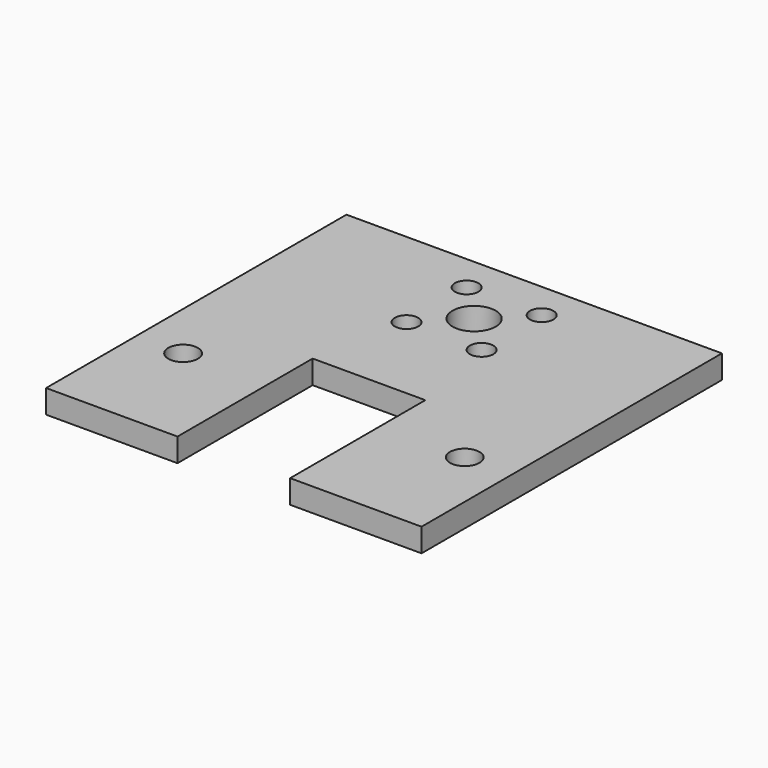
from build123d import *

# Parameters (mm, degrees)
F0_R     = 2
F0_R_2   = 1.5875
F0_R_3   = 2.921
F1_DEPTH = 3.175


# Not quite as in the source:
# - a feature names something its author has since deleted; it is built from what else it names


with BuildPart() as f1:
    # F0 (on Top) → F1 (new body)
    with BuildSketch(Plane.XY):
        Polygon((-25.4, 76.2436284547), (-25.4, 25.4436284547), (-7.62, 25.4436284547), (-7.62, 48.3036284547), (7.62, 48.3036284547), (7.62, 25.4436284547), (25.4, 25.4436284547), (25.4, 76.2436284547), align=None)
        with Locations((-19.05, 40.6836284547)):
            Circle(F0_R, mode=Mode.SUBTRACT)
        with Locations((19.05, 40.6836284547)):
            Circle(F0_R, mode=Mode.SUBTRACT)
        with Locations((-5.08, 61.0036284547)):
            Circle(F0_R_2, mode=Mode.SUBTRACT)
        with Locations((0, 66.0836284547)):
            Circle(F0_R_3, mode=Mode.SUBTRACT)
        with Locations((-5.08, 71.1636284547)):
            Circle(F0_R_2, mode=Mode.SUBTRACT)
        with Locations((5.08, 61.0036284547)):
            Circle(F0_R_2, mode=Mode.SUBTRACT)
        with Locations((5.08, 71.1636284547)):
            Circle(F0_R_2, mode=Mode.SUBTRACT)
    extrude(amount=F1_DEPTH)


solid = f1.part
